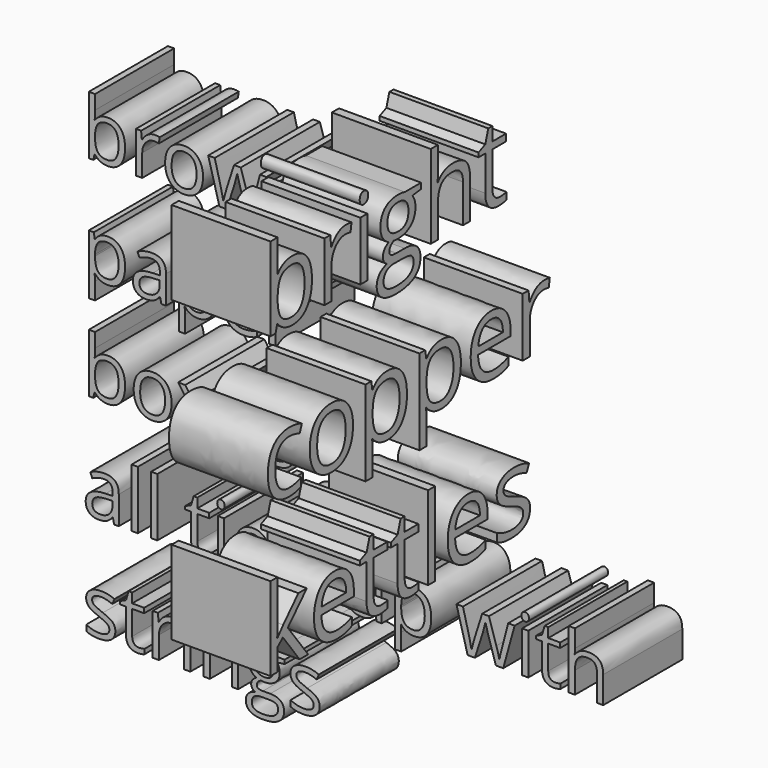
from build123d import *

# Parameters (mm, degrees)
F0_TEXT_SIZE = 28.2443594187
F1_DEPTH     = 25.4
F2_TEXT_SIZE = 19.784235499
F3_DEPTH     = 25.4


# Not quite as in the source:
# - Text() gives the source's letters only with a copy of the font that has no kerning and outlines rounded to 1/6400 em; it was checked with that copy


with BuildPart() as f1:
    # F0 (on Right) → F1 (new body)
    with BuildSketch(Plane.YZ):
        with Locations((-77.7523219585, 43.8503064215)):
            Text('bright', F0_TEXT_SIZE, font='Open Sans', text_align=(TextAlign.LEFT, TextAlign.BOTTOM))
        with Locations((-77.7523219585, 5.437977612)):
            Text('copper', F0_TEXT_SIZE, font='Open Sans', text_align=(TextAlign.LEFT, TextAlign.BOTTOM))
        with Locations((-77.7523219585, -32.9743511975)):
            Text('kettles', F0_TEXT_SIZE, font='Open Sans', text_align=(TextAlign.LEFT, TextAlign.BOTTOM))
    extrude(amount=F1_DEPTH)


with BuildPart() as f3:
    # F2 (on Front) → F3 (new body)
    with BuildSketch(Plane.XZ):
        with Locations((-62.9205182195, 35.6798805296)):
            Text('brown', F2_TEXT_SIZE, font='Open Sans', text_align=(TextAlign.LEFT, TextAlign.BOTTOM))
        with Locations((-62.9205182195, 8.773320251)):
            Text('paper', F2_TEXT_SIZE, font='Open Sans', text_align=(TextAlign.LEFT, TextAlign.BOTTOM))
        with Locations((-62.9205182195, -18.1332400276)):
            Text('boxes', F2_TEXT_SIZE, font='Open Sans', text_align=(TextAlign.LEFT, TextAlign.BOTTOM))
        with Locations((-62.9205182195, -45.0398003062)):
            Text('all tied up with', F2_TEXT_SIZE, font='Open Sans', text_align=(TextAlign.LEFT, TextAlign.BOTTOM))
        with Locations((-62.9205182195, -71.9463605848)):
            Text('strings', F2_TEXT_SIZE, font='Open Sans', text_align=(TextAlign.LEFT, TextAlign.BOTTOM))
    extrude(amount=F3_DEPTH)


solid = Compound([f1.part, f3.part])
